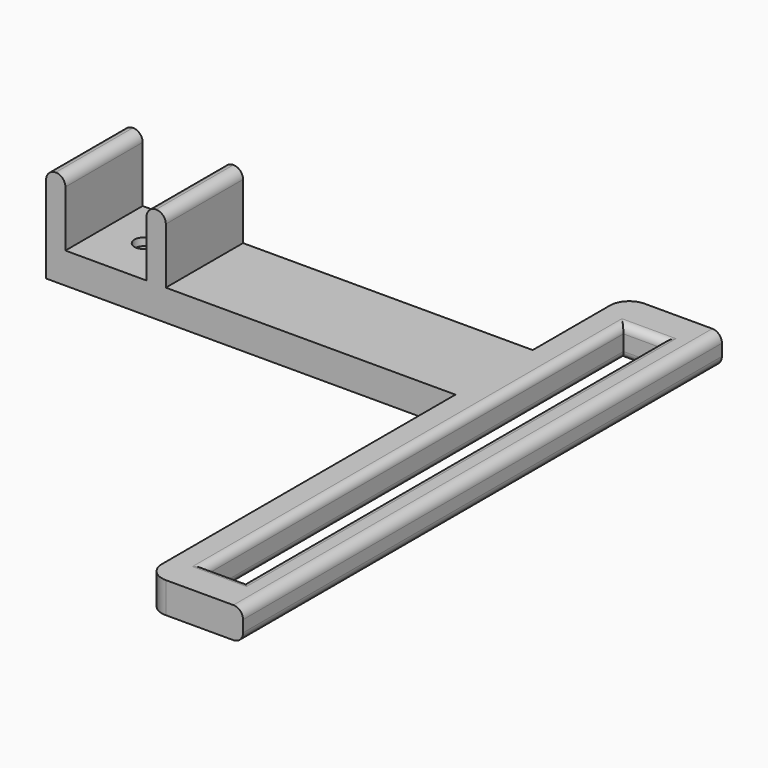
from build123d import *

# Parameters (mm, degrees)
F0_W      = 5
F0_H      = 17
F0_H_2    = 8
F0_W_2    = 21
F0_W_3    = 100
F1_DEPTH  = 25
F3_DEPTH  = 8
F4_R      = 2.5
F5_R      = 2.49999
F6_R      = 2.6
F7_DEPTH  = 25
F8_R      = 5
F9_R      = 4.5
F9_R_2    = 2.6
F10_DEPTH = 6
F2_W      = 10
F2_H      = 25
F11_DEPTH = 25
F12_R     = 2


# Not quite as in the source:
# - a fillet or chamfer is up to 0.001 mm smaller than in the source, because OpenCascade refuses the exact size


with BuildPart() as f1:
    # F0 (on Front) → F1 (new body)
    with BuildSketch(Plane.XZ):
        with Locations((-16.2189533483, 16.5)):
            Rectangle(F0_W, F0_H)
        with Locations((-16.2189533483, 4)):
            Rectangle(F0_W, F0_H_2)
        with Locations((-3.2189533483, 4)):
            Rectangle(F0_W_2, F0_H_2)
        with Locations((9.7810466517, 4)):
            Rectangle(F0_W, F0_H_2)
        with Locations((9.7810466517, 16.5)):
            Rectangle(F0_W, F0_H)
        with Locations((62.2810466517, 4)):
            Rectangle(F0_W_3, F0_H_2)
    extrude(amount=F1_DEPTH)

    # F2 (on face) → F3 (join)
    with BuildSketch(Plane.XY.offset(8)):
        Polygon((87.2810466517, -125), (112.2810466517, -125), (112.2810466517, -25), (104.7810466517, -25), (104.7810466517, -115), (94.7810466517, -115), (94.7810466517, -25), (87.2810466517, -25), align=None)
        Polygon((104.7810466517, 0), (112.2810466517, 0), (112.2810466517, 30), (87.2810466517, 30), (87.2810466517, 0), (94.7810466517, 0), (94.7810466517, 20), (104.7810466517, 20), align=None)
    extrude(amount=-F3_DEPTH)

    # F4
    f4_edges = [f1.edges().sort_by_distance(p)[0] for p in [
        (112.281047, -47.5, 0),
        (112.281047, -47.5, 8),
    ]]
    fillet(f4_edges, radius=F4_R)

    # F5 (radius 2.5 in the source; OpenCascade refuses exactly that, so slightly less here)
    f5_edges = [f1.edges().sort_by_distance(p)[0] for p in [
        (12.281047, -12.5, 25),
        (7.281047, -12.5, 25),
        (-18.718953, -12.5, 25),
        (-13.718953, -12.5, 25),
    ]]
    fillet(f5_edges, radius=F5_R)

    # F6 (on face) → F7 (cut)
    with BuildSketch(Plane.XY.offset(8)):
        with Locations((-3.2189533483, -12.5)):
            Circle(F6_R)
    extrude(amount=-F7_DEPTH, mode=Mode.SUBTRACT)

    # F8
    f8_edges = [f1.edges().sort_by_distance(p)[0] for p in [
        (87.281047, 30, 4),
        (87.281047, -125, 4),
    ]]
    fillet(f8_edges, radius=F8_R)

    # F9 (on face) → F10 (cut)
    with BuildSketch(Plane(origin=(0, 0, 0), x_dir=(1, 0, 0), z_dir=(0, 0, -1))):
        with Locations((-3.2189533483, 12.5)):
            Circle(F9_R)
        with Locations((-3.2189533483, 12.5)):
            Circle(F9_R_2, mode=Mode.SUBTRACT)
    extrude(amount=-F10_DEPTH, mode=Mode.SUBTRACT)

    # F2 (on face) → F11 (cut)
    with BuildSketch(Plane.XY.offset(8)):
        with Locations((99.7810466517, -12.5)):
            Rectangle(F2_W, F2_H)
    extrude(amount=-F11_DEPTH, mode=Mode.SUBTRACT)

    # F12
    f12_edges = [f1.edges().sort_by_distance(p)[0] for p in [
        (94.781047, -47.5, 8),
        (99.781047, 20, 8),
        (104.781047, -47.5, 8),
        (99.781047, -115, 8),
        (99.781047, 20, 0),
        (94.781047, -47.5, 0),
        (104.781047, -47.5, 0),
        (99.781047, -115, 0),
    ]]
    fillet(f12_edges, radius=F12_R)


solid = f1.part
